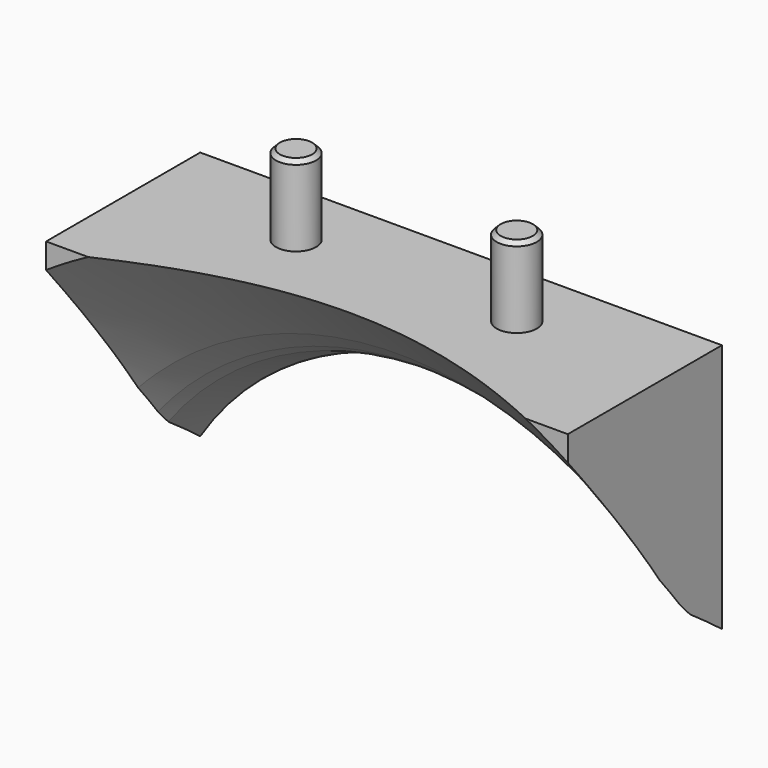
from build123d import *

# Parameters (mm, degrees)
F1_DEPTH    = 60.96
F2_T2_ANGLE = 359.64
F3_SIZE     = 10.15999
F4_R        = 6.35
F5_DEPTH    = 25.4
F6_SIZE     = 1.27
F7_SIZE     = 5.08
F8_SIZE     = 5.08


# Not quite as in the source:
# - a fillet or chamfer that OpenCascade refuses, or shapes differently, is made with other operations: its cross-section is extruded or revolved along the edge and cut away or added
# - a fillet or chamfer is up to 0.001 mm smaller than in the source, because OpenCascade refuses the exact size


with BuildPart() as f1:
    # F0 (on Front) → F1 (new body)
    with BuildSketch(Plane.XZ):
        with BuildLine():
            Line((68.6990445861, 54.4476021031), (0, 54.4476021031))
            Line((0, 54.4476021031), (-96.4009554139, 54.4476021031))
            Line((-96.4009554139, 54.4476021031), (-96.4009554139, -24.6122339721))
            ThreePointArc((-96.4009554139, -24.6122339721), (-13.8509554139, 20.7245603096), (68.6990445861, -24.6122339721))
            Line((68.6990445861, -24.6122339721), (68.6990445861, 54.4476021031))
        make_face()
    extrude(amount=F1_DEPTH)

    # F2: chamfer of 50.8 on 1 edges, made by hand

    # F2_s1 → F2_t2 (revolve, cut)
    with BuildSketch(Plane(origin=(-13.6086096269, 0, 0.0427528487), x_dir=(0, 1, 0), z_dir=(0.9999950652, 0, -0.0031415875))):
        Polygon((-60.96, -225.7638003707), (-10.16, -174.9638003707), (-60.96, -174.9638003707), align=None)
    revolve(axis=Axis((-13.8509554139, -60.96, -77.0980532681), (0, 1, 0)), revolution_arc=F2_T2_ANGLE, mode=Mode.SUBTRACT)

    # F3 (size 10.16 in the source; OpenCascade refuses exactly that, so slightly less here)
    f3_edges = [f1.edges().sort_by_distance(p)[0] for p in [
        (-13.850955, -10.16, 20.72456),
    ]]
    chamfer(f3_edges, length=F3_SIZE)

    # F4 (on face) → F5 (join)
    with BuildSketch(Plane.XY.offset(54.4476021031)):
        with Locations((-48.7759554139, -21.6264873743)):
            Circle(F4_R)
        with Locations((21.0740445861, -21.6264873743)):
            Circle(F4_R)
    extrude(amount=F5_DEPTH)

    # F6
    f6_edges = [f1.edges().sort_by_distance(p)[0] for p in [
        (-55.125955, -21.626487, 79.847602),
        (14.724045, -21.626487, 79.847602),
    ]]
    chamfer(f6_edges, length=F6_SIZE)

    # F7
    f7_edges = [f1.edges().sort_by_distance(p)[0] for p in [
        (-13.850955, -17.344239, 27.9088),
    ]]
    chamfer(f7_edges, length=F7_SIZE)

    # F8
    f8_edges = [f1.edges().sort_by_distance(p)[0] for p in [
        (-13.850955, -20.936342, 31.500902),
    ]]
    chamfer(f8_edges, length=F8_SIZE)


solid = f1.part
